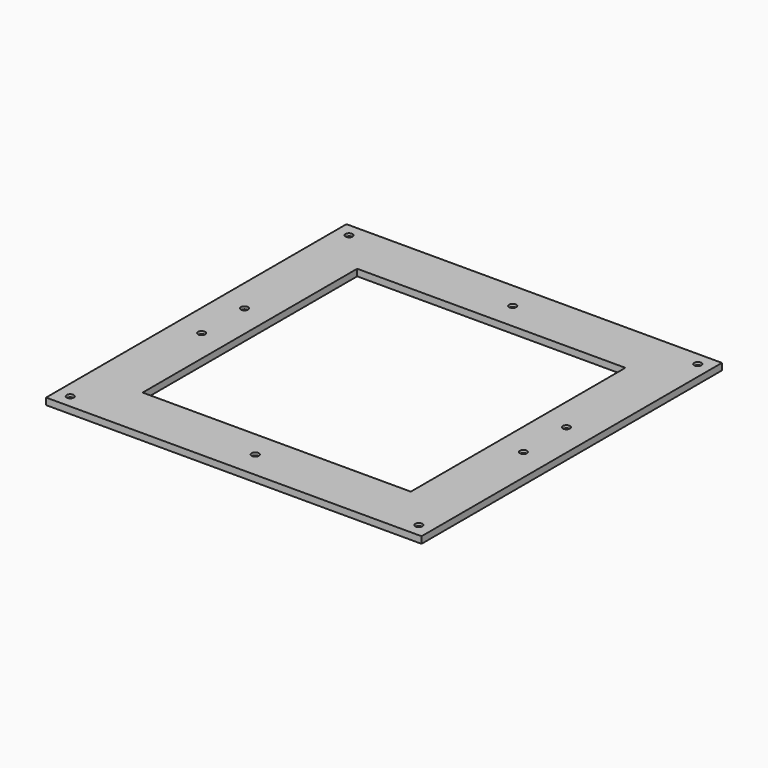
from build123d import *

# Parameters (mm, degrees)
F0_W           = 355.6
F0_H           = 355.6
F0_W_2         = 254
F0_H_2         = 254
F1_DEPTH       = 6.35
F2_D           = 6.7564
F2_DEPTH       = 26.0604
F2_CSINK_D     = 13.4874
F2_CSINK_ANGLE = 82
F2_TIP         = 2.0298273432


# Not quite as in the source:
# - a feature names something its author has since deleted; it is built from what else it names


with BuildPart() as f1:
    # F0 (on Top) → F1 (new body)
    with BuildSketch(Plane.XY):
        with Locations((177.8, 177.8)):
            Rectangle(F0_W, F0_H)
        with Locations((177.8, 177.8)):
            Rectangle(F0_W_2, F0_H_2, mode=Mode.SUBTRACT)
    extrude(amount=F1_DEPTH)

    # F2
    with Locations(Plane(origin=(0, 0, 0), x_dir=(1, 0, 0), z_dir=(0, 0, -1))):
        with Locations((12.7, -342.9), (342.9, -342.9), (342.9, -12.7), (12.7, -12.7), (177.8, -25.4), (177.8, -330.2), (25.4, -152.4), (330.2, -203.2), (330.2, -152.4), (25.4, -203.2)):
            CounterSinkHole(F2_D / 2, F2_CSINK_D / 2, depth=F2_DEPTH, counter_sink_angle=F2_CSINK_ANGLE)
            with Locations((0, 0, -(F2_DEPTH + F2_TIP / 2))):  # 118° drill point
                Cone(0, F2_D / 2, F2_TIP, mode=Mode.SUBTRACT)


solid = f1.part
